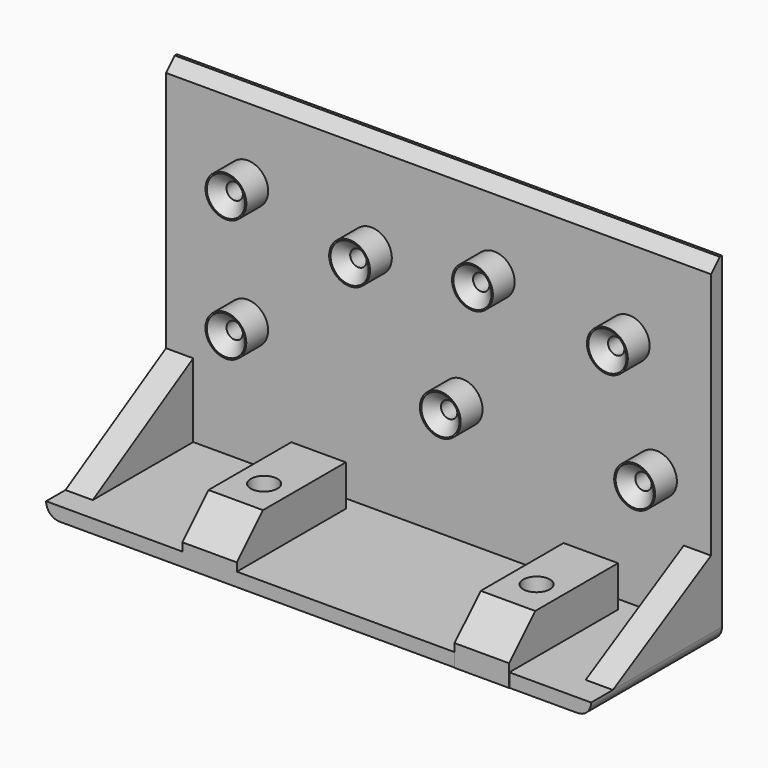
from build123d import *

# Parameters (mm, degrees)
F1_W      = 127
F1_H      = 38.1
F2_DEPTH  = 3.175
F4_W      = 127
F4_H      = 3.175
F5_DEPTH  = 76.2
F7_W      = 12.7
F7_H      = 31.75
F8_DEPTH  = 12.7
F6_R      = 2.667
F9_DEPTH  = 25.4
F9_TAPER  = -2
F10_R     = 3.17499
F12_DEPTH = 6.35
F14_DEPTH = 6.35
F15_R     = 4.7625
F16_DEPTH = 6.35
F17_R     = 1.905
F18_DEPTH = 25.4
F19_SIZE  = 2.54
F20_SIZE  = 2.54
F21_SIZE  = 7.62


# Not quite as in the source:
# - a fillet or chamfer is up to 0.001 mm smaller than in the source, because OpenCascade refuses the exact size


with BuildPart() as f2:
    # F1 (on Top) → F2 (new body)
    with BuildSketch(Plane.XY):
        with Locations((63.5, -19.05)):
            Rectangle(F1_W, F1_H)
    extrude(amount=F2_DEPTH)

    # F4 (on face) → F5 (join)
    with BuildSketch(Plane.XY.offset(3.175)):
        with Locations((63.5, -1.5875)):
            Rectangle(F4_W, F4_H)
    extrude(amount=F5_DEPTH)

    # F7 (on Top) → F8 (join)
    with BuildSketch(Plane.XY):
        with Locations((38.1, -22.225)):
            Rectangle(F7_W, F7_H)
        with Locations((101.6, -22.3082778975)):
            Rectangle(F7_W, F7_H)
    extrude(amount=F8_DEPTH)

    # F6 (on Top) → F9 (cut)
    with BuildSketch(Plane.XY):
        with Locations((38.1, -22.225)):
            Circle(F6_R)
        with Locations((101.6, -22.225)):
            Circle(F6_R)
    extrude(amount=F9_DEPTH, taper=F9_TAPER, mode=Mode.SUBTRACT)

    # F10 (radius 3.175 in the source; OpenCascade refuses exactly that, so slightly less here)
    f10_edges = [f2.edges().sort_by_distance(p)[0] for p in [
        (0, -19.05, 0),
        (127, -19.05, 0),
    ]]
    fillet(f10_edges, radius=F10_R)

    # F11 (on face) → F12 (join)
    with BuildSketch(Plane(origin=(0, 0, 0), x_dir=(0, -1, 0), z_dir=(-1, 0, 0))):
        Polygon((32.4499383569, 3.175), (0, 22.225), (0, 3.175), align=None)
    extrude(amount=-F12_DEPTH)

    # F13 (on face) → F14 (join)
    with BuildSketch(Plane.YZ.offset(127)):
        Polygon((0, 3.175), (0, 20.8942663938), (-31.75, 3.175), align=None)
    extrude(amount=-F14_DEPTH)

    # F15 (on face) → F16 (join)
    with BuildSketch(Plane.XZ.offset(3.175)):
        with Locations((19.05, 60.3252180792)):
            Circle(F15_R)
        with Locations((47.8610846677, 55.9717772163)):
            Circle(F15_R)
        with Locations((76.4872658529, 60.3252180792)):
            Circle(F15_R)
        with Locations((107.9343466558, 57.469660566)):
            Circle(F15_R)
        with Locations((19.0343466558, 31.75)):
            Circle(F15_R)
        with Locations((69.0070766487, 31.75)):
            Circle(F15_R)
        with Locations((114.2843466558, 31.75)):
            Circle(F15_R)
    extrude(amount=F16_DEPTH)

    # F17 (on Front) → F18 (cut)
    with BuildSketch(Plane.XZ):
        with Locations((19.05, 60.325)):
            Circle(F17_R)
        with Locations((47.8767380118, 55.9715591371)):
            Circle(F17_R)
        with Locations((76.5029191971, 60.325)):
            Circle(F17_R)
        with Locations((107.95, 57.4694424868)):
            Circle(F17_R)
        with Locations((19.05, 31.75)):
            Circle(F17_R)
        with Locations((69.0227299929, 31.75)):
            Circle(F17_R)
        with Locations((114.3, 31.75)):
            Circle(F17_R)
    extrude(amount=F18_DEPTH, mode=Mode.SUBTRACT)

    # F19
    f19_edges = [f2.edges().sort_by_distance(p)[0] for p in [
        (17.145, -9.525, 60.325),
        (45.971738, -9.525, 55.971559),
        (74.597919, -9.525, 60.325),
        (17.145, -9.525, 31.75),
        (106.045, -9.525, 57.469442),
        (112.395, -9.525, 31.75),
        (67.11773, -9.525, 31.75),
    ]]
    chamfer(f19_edges, length=F19_SIZE)

    # F20
    f20_edges = [f2.edges().sort_by_distance(p)[0] for p in [
        (63.5, -3.175, 79.375),
    ]]
    chamfer(f20_edges, length=F20_SIZE)

    # F21
    f21_edges = [f2.edges().sort_by_distance(p)[0] for p in [
        (38.1, -38.1, 12.7),
        (101.6, -38.183278, 12.7),
    ]]
    chamfer(f21_edges, length=F21_SIZE)


solid = f2.part
